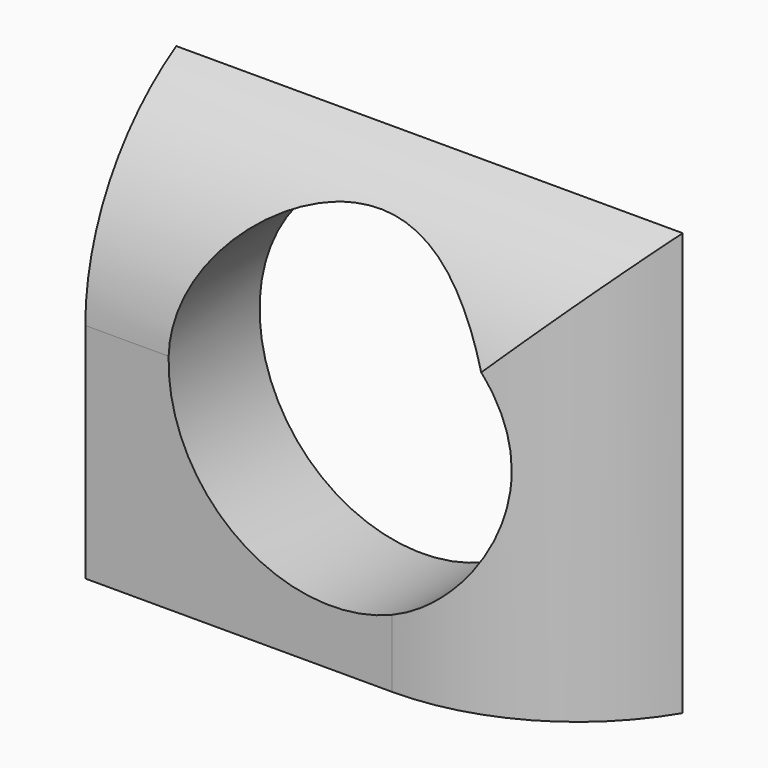
from build123d import *

# Parameters (mm, degrees)
F0_W        = 111.2626455724
F0_H        = 92.8305797279
F0_R        = 35.6593077027
F1_DEPTH    = 25
F2_T1_DEPTH = 312.2046894127
F2_T3_DEPTH = 330.6367552572


# Not quite as in the source:
# - a fillet or chamfer that OpenCascade refuses, or shapes differently, is made with other operations: its cross-section is extruded or revolved along the edge and cut away or added


with BuildPart() as f1:
    # F0 (on Front) → F1 (new body)
    with BuildSketch(Plane.XZ):
        with Locations((1.6756337136, -1.5080738813)):
            Rectangle(F0_W, F0_H)
        Circle(F0_R, mode=Mode.SUBTRACT)
    extrude(amount=F1_DEPTH)

    # F2: fillet of radius 51 on 2 edges, made by hand

    # F2_s2 → F2_t1 (cut)
    with BuildSketch(Plane.XY.offset(-157.6104185876)):
        with BuildLine():
            ThreePointArc((57.3069564998, 0), (38.6808969088, -18.3113980822), (13.4321345628, -25))
            Line((13.4321345628, -25), (57.3069564998, -25))
            Line((57.3069564998, -25), (57.3069564998, 0))
        make_face()
    extrude(amount=F2_T1_DEPTH, mode=Mode.SUBTRACT)

    # F2_s4 → F2_t3 (cut)
    with BuildSketch(Plane.YZ.offset(-163.642743915)):
        with BuildLine():
            ThreePointArc((0, 44.9072159827), (-18.3113980822, 26.2811563916), (-25, 1.0323940457))
            Line((-25, 1.0323940457), (-25, 44.9072159827))
            Line((-25, 44.9072159827), (0, 44.9072159827))
        make_face()
    extrude(amount=F2_T3_DEPTH, mode=Mode.SUBTRACT)


solid = f1.part
